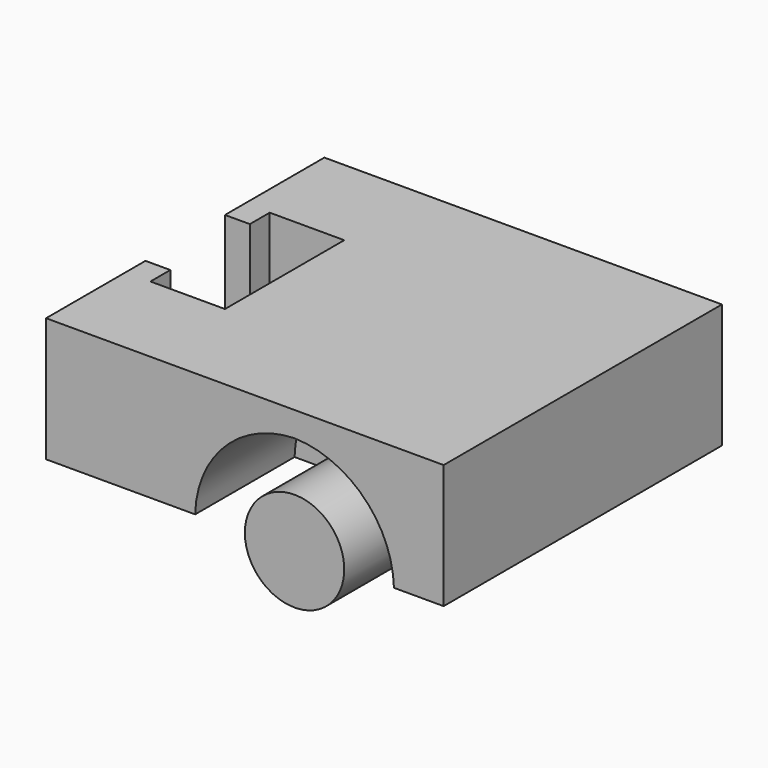
from build123d import *

# Parameters (mm, degrees)
F0_W          = 70
F0_H          = 25
F1_DEPTH      = 40
F1_DEPTH_BACK = 40
F3_DEPTH      = 40
F4_W          = 40
F4_H          = 20
F5_DEPTH      = 25
F7_DEPTH      = 25
F8_W          = 80
F8_H          = 25
F9_DEPTH      = 35
F11_DEPTH     = 25
F12_T4_DEPTH  = 76.2347538298
F12_T9_DEPTH  = 76.2347538298
F12_T14_DEPTH = 76.2347538298
F12_T19_DEPTH = 76.2347538298


# Not quite as in the source:
# - a fillet or chamfer that OpenCascade refuses, or shapes differently, is made with other operations: its cross-section is extruded or revolved along the edge and cut away or added


with BuildPart() as f1:
    # F0 (on Right) → F1 (new body, two sides)
    with BuildSketch(Plane.YZ) as f1_sk:
        Rectangle(F0_W, F0_H)
    extrude(amount=F1_DEPTH)
    extrude(f1_sk.sketch, amount=-F1_DEPTH_BACK)

    # F2 (on face) → F3 (cut)
    with BuildSketch(Plane.XY.offset(12.5)):
        Polygon((-40, 10), (-40, 0), (-20, 0), (-20, 15), (-35, 15), (-35, 10), align=None)
        Polygon((-20, 0), (-40, 0), (-40, -10), (-35, -10), (-35, -15), (-20, -15), align=None)
    extrude(amount=-F3_DEPTH, mode=Mode.SUBTRACT)

    # F4 (on face) → F5 (cut)
    with BuildSketch(Plane.XZ.offset(35)):
        with Locations((10, -2.5)):
            Rectangle(F4_W, F4_H)
    extrude(amount=-F5_DEPTH, mode=Mode.SUBTRACT)

    # F6 (on face) → F7 (join)
    with BuildSketch(Plane.XZ.offset(10)):
        with BuildLine():
            Line((0, -12.5), (20, -12.5))
            ThreePointArc((20, -12.5), (10, -2.5), (0, -12.5))
        make_face()
        with BuildLine():
            ThreePointArc((0, -12.5), (10, -22.5), (20, -12.5))
            Line((20, -12.5), (0, -12.5))
        make_face()
    extrude(amount=F7_DEPTH)

    # F8 (on face) → F9 (cut)
    with BuildSketch(Plane(origin=(0, 35, 0), x_dir=(-1, 0, 0), z_dir=(0, 1, 0))):
        Rectangle(F8_W, F8_H)
    extrude(amount=-F9_DEPTH, mode=Mode.SUBTRACT)

    # F10: F1 across plane


with BuildPart() as f1_1:
    add(f1.part)
    add(f1.part.mirror(Plane.XZ))

    # F11 (add): a face of the model
    f11_faces = [f1_1.faces().sort_by_distance(p)[0] for p in [
        (10, -10, -16.7441318158),
    ]]
    extrude(f11_faces, amount=F11_DEPTH)

    # F12: fillet of radius 20.5 on 4 edges, made by hand


with BuildPart() as f12_tool2:
    # F12_s3 → F12_t4 (new body)
    with BuildSketch(Plane.XZ.offset(-35)):
        with BuildLine():
            ThreePointArc((30, -12.5), (23.8239195314, 1.6714007511), (9.5060984681, 7.5))
            Line((9.5060984681, 7.5), (30, 7.5))
            Line((30, 7.5), (30, -12.5))
        make_face()
    extrude(amount=F12_T4_DEPTH)

    split(bisect_by=Plane.XZ.offset(35), keep=Keep.BOTTOM)


with BuildPart() as f1_2:
    add(f1_1.part)

    # F12_t1: union F12_tool2
    add(f12_tool2.part)


with BuildPart() as f12_tool7:
    # F12_s8 → F12_t9 (new body)
    with BuildSketch(Plane.XZ.offset(-35)):
        with BuildLine():
            ThreePointArc((10.4939015319, 7.5), (-3.8239195314, 1.6714007511), (-10, -12.5))
            Line((-10, -12.5), (-10, 7.5))
            Line((-10, 7.5), (10.4939015319, 7.5))
        make_face()
    extrude(amount=F12_T9_DEPTH)

    split(bisect_by=Plane.XZ.offset(35), keep=Keep.BOTTOM)


with BuildPart() as f1_3:
    add(f1_2.part)

    # F12_t6: union F12_tool7
    add(f12_tool7.part)


with BuildPart() as f12_tool12:
    # F12_s13 → F12_t14 (new body)
    with BuildSketch(Plane.XZ.offset(35)):
        with BuildLine():
            ThreePointArc((30, -12.5), (23.8239195314, 1.6714007511), (9.5060984681, 7.5))
            Line((9.5060984681, 7.5), (30, 7.5))
            Line((30, 7.5), (30, -12.5))
        make_face()
    extrude(amount=-F12_T14_DEPTH)

    split(bisect_by=Plane.XZ.offset(-35), keep=Keep.TOP)


with BuildPart() as f1_4:
    add(f1_3.part)

    # F12_t11: union F12_tool12
    add(f12_tool12.part)


with BuildPart() as f12_tool17:
    # F12_s18 → F12_t19 (new body)
    with BuildSketch(Plane.XZ.offset(35)):
        with BuildLine():
            ThreePointArc((-10, -12.5), (-3.8239195314, 1.6714007511), (10.4939015319, 7.5))
            Line((10.4939015319, 7.5), (-10, 7.5))
            Line((-10, 7.5), (-10, -12.5))
        make_face()
    extrude(amount=-F12_T19_DEPTH)

    split(bisect_by=Plane.XZ.offset(-35), keep=Keep.TOP)


with BuildPart() as f1_5:
    add(f1_4.part)

    # F12_t16: union F12_tool17
    add(f12_tool17.part)


solid = f1_5.part
